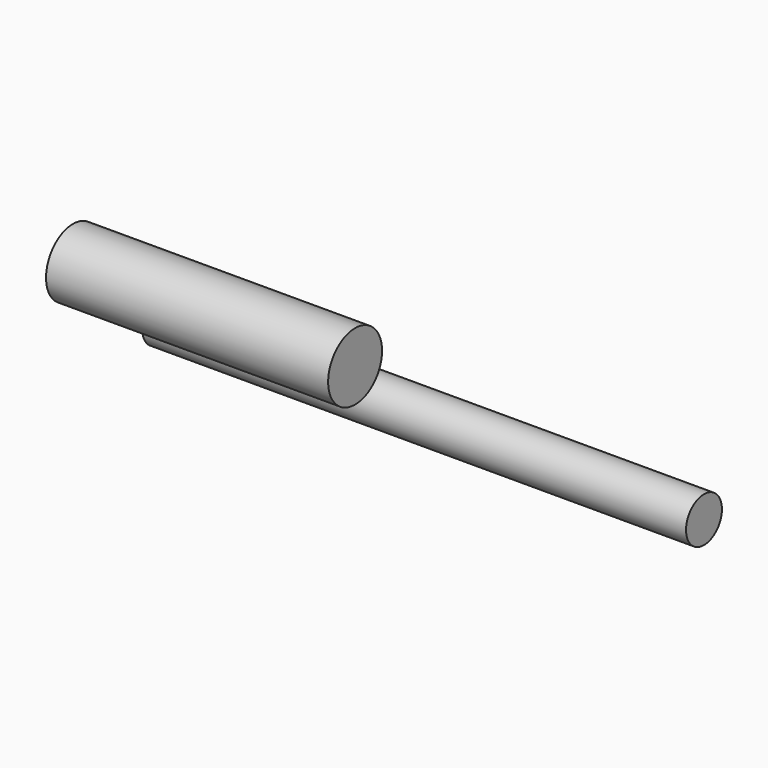
from build123d import *

# Parameters (mm, degrees)
F0_R     = 48.4684521976
F3_DEPTH = 1175.004
F2_R     = 72.7943383902
F4_DEPTH = 609.6


# Not quite as in the source:
# - the program builds the solid bodies; features that only make, move or delete a surface that nothing else refers to are left out


with BuildPart() as f3:
    # F0 (on Right) → F3 (new body)
    with BuildSketch(Plane.YZ):
        with Locations((172.7738380432, 15.8285461366)):
            Circle(F0_R)
    extrude(amount=F3_DEPTH)


with BuildPart() as f4:
    # F2 (on Right) → F4 (new body)
    with BuildSketch(Plane.YZ):
        with Locations((-62.7910271287, 219.3149775267)):
            Circle(F2_R)
    extrude(amount=F4_DEPTH)


solid = Compound([f3.part, f4.part])
